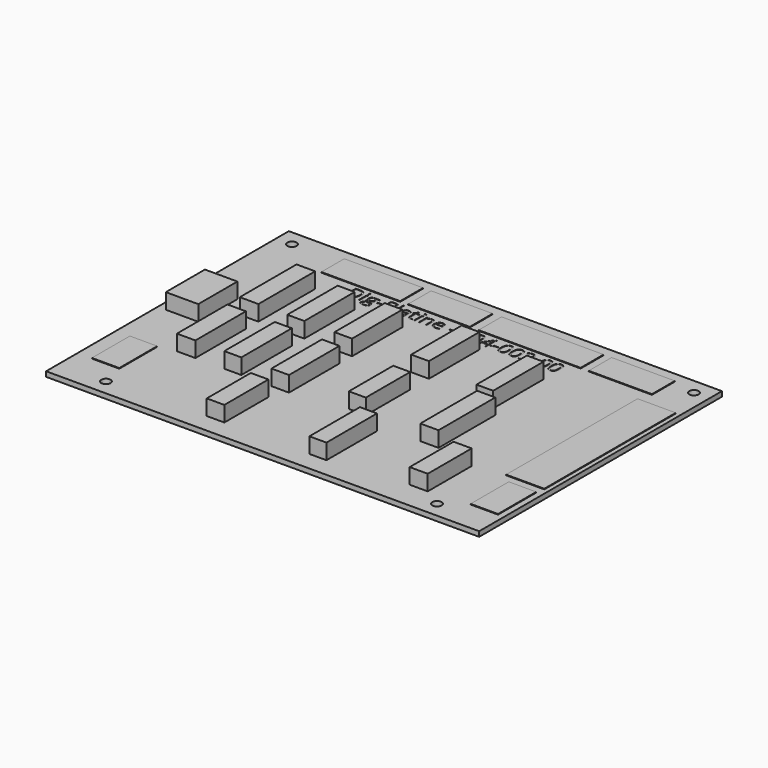
from build123d import *

# Parameters (mm, degrees)
F0_W         = 139.5791522491
F0_H         = 97.79
F0_R         = 1.5
F0_W_2       = 8.8093318045
F0_H_2       = 15.2748934925
F0_W_3       = 5.6705586612
F0_H_3       = 17.7562497556
F0_W_4       = 5.9523582458
F0_H_4       = 20.3446323285
F0_W_5       = 5.4862108082
F0_W_6       = 5.6576561183
F0_W_7       = 5.4957289249
F0_H_5       = 20.3665252775
F0_W_8       = 5.819004029
F0_H_6       = 17.6994800568
F0_W_9       = 8.8422298431
F0_H_7       = 15.3777878731
F0_W_10      = 5.4677436128
F0_H_8       = 17.8766759345
F0_W_11      = 5.862781778
F0_H_9       = 22.8744579945
F0_W_12      = 10.4659721255
F0_H_10      = 15.7669195905
F0_W_13      = 6.0005448759
F0_H_11      = 22.8592171334
F0_H_12      = 20.2875542454
F0_W_14      = 25.4173632711
F0_H_13      = 9.2426761985
F0_W_15      = 19.8445699643
F0_W_16      = 5.7087126188
F0_H_14      = 20.3202972189
F0_W_17      = 5.3689070046
F0_W_18      = 12.3022273183
F0_H_15      = 52.9572535306
F0_W_19      = 32.893058029
F0_W_20      = 20.3882530332
F1_DEPTH     = 1.6
F2_TEXT_SIZE = 6.1743944469
F3_DEPTH     = 0.1
F4_DEPTH     = 0.2
F5_DEPTH     = 5


# Not quite as in the source:
# - Text() gives the source's letters only with a copy of the font that has no kerning and outlines rounded to 1/6400 em; it was checked with that copy


with BuildPart() as f1:
    # F0 (on Top) → F1 (new body)
    with BuildSketch(Plane.XY):
        Rectangle(F0_W, F0_H)
        with Locations((-54.5495761246, -43.815)):
            Circle(F0_R, mode=Mode.SUBTRACT)
        with Locations((-60.6642495841, -28.6812912673)):
            Rectangle(F0_W_2, F0_H_2, mode=Mode.SUBTRACT)
        with Locations((-20.1366990805, -33.8139589876)):
            Rectangle(F0_W_3, F0_H_3, mode=Mode.SUBTRACT)
        with Locations((-47.9160919785, -9.6386900987)):
            Rectangle(F0_W_4, F0_H_4, mode=Mode.SUBTRACT)
        with Locations((-32.8816743568, -9.6386900987)):
            Rectangle(F0_W_5, F0_H_4, mode=Mode.SUBTRACT)
        with Locations((-17.594573088, -9.6386900987)):
            Rectangle(F0_W_6, F0_H_4, mode=Mode.SUBTRACT)
        with Locations((12.853551656, -32.5088212267)):
            Rectangle(F0_W_7, F0_H_5, mode=Mode.SUBTRACT)
        with Locations((52.1304238754, -43.815)):
            Circle(F0_R, mode=Mode.SUBTRACT)
        with Locations((43.2012882084, -31.1752967536)):
            Rectangle(F0_W_8, F0_H_6, mode=Mode.SUBTRACT)
        with Locations((63.4397342801, -31.1942892149)):
            Rectangle(F0_W_9, F0_H_7, mode=Mode.SUBTRACT)
        with Locations((5.2794092335, -8.4047119017)):
            Rectangle(F0_W_10, F0_H_8, mode=Mode.SUBTRACT)
        with Locations((30.4834870622, -8.3737772657)):
            Rectangle(F0_W_11, F0_H_9, mode=Mode.SUBTRACT)
        with Locations((-61.9684271514, 3.9792419411)):
            Rectangle(F0_W_12, F0_H_10, mode=Mode.SUBTRACT)
        with Locations((-47.9401852936, 17.0108985621)):
            Rectangle(F0_W_13, F0_H_11, mode=Mode.SUBTRACT)
        with Locations((-32.8816743568, 15.7250671182)):
            Rectangle(F0_W_5, F0_H_12, mode=Mode.SUBTRACT)
        with Locations((-17.594573088, 15.7250671182)):
            Rectangle(F0_W_6, F0_H_12, mode=Mode.SUBTRACT)
        with Locations((-64.7095761246, 43.815)):
            Circle(F0_R, mode=Mode.SUBTRACT)
        with Locations((-36.5455234423, 40.930185467)):
            Rectangle(F0_W_14, F0_H_13, mode=Mode.SUBTRACT)
        with Locations((-11.3320440287, 40.930185467)):
            Rectangle(F0_W_15, F0_H_13, mode=Mode.SUBTRACT)
        with Locations((5.1589247305, 18.2475312613)):
            Rectangle(F0_W_16, F0_H_14, mode=Mode.SUBTRACT)
        with Locations((28.0277524143, 15.7250671182)):
            Rectangle(F0_W_17, F0_H_12, mode=Mode.SUBTRACT)
        with Locations((62.2001700103, 5.6103980169)):
            Rectangle(F0_W_18, F0_H_15, mode=Mode.SUBTRACT)
        with Locations((17.8911256953, 40.930185467)):
            Rectangle(F0_W_19, F0_H_13, mode=Mode.SUBTRACT)
        with Locations((47.1142940223, 40.930185467)):
            Rectangle(F0_W_20, F0_H_13, mode=Mode.SUBTRACT)
        with Locations((64.8304238754, 43.815)):
            Circle(F0_R, mode=Mode.SUBTRACT)
        with Locations((-36.5455234423, 40.930185467)):
            Rectangle(F0_W_14, F0_H_13)
        with Locations((-11.3320440287, 40.930185467)):
            Rectangle(F0_W_15, F0_H_13)
        with Locations((17.8911256953, 40.930185467)):
            Rectangle(F0_W_19, F0_H_13)
        with Locations((47.1142940223, 40.930185467)):
            Rectangle(F0_W_20, F0_H_13)
        with Locations((-47.9401852936, 17.0108985621)):
            Rectangle(F0_W_13, F0_H_11)
        with Locations((-32.8816743568, 15.7250671182)):
            Rectangle(F0_W_5, F0_H_12)
        with Locations((-17.594573088, 15.7250671182)):
            Rectangle(F0_W_6, F0_H_12)
        with Locations((5.1589247305, 18.2475312613)):
            Rectangle(F0_W_16, F0_H_14)
        with Locations((28.0277524143, 15.7250671182)):
            Rectangle(F0_W_17, F0_H_12)
        with Locations((62.2001700103, 5.6103980169)):
            Rectangle(F0_W_18, F0_H_15)
        with Locations((-61.9684271514, 3.9792419411)):
            Rectangle(F0_W_12, F0_H_10)
        with Locations((-47.9160919785, -9.6386900987)):
            Rectangle(F0_W_4, F0_H_4)
        with Locations((-32.8816743568, -9.6386900987)):
            Rectangle(F0_W_5, F0_H_4)
        with Locations((-17.594573088, -9.6386900987)):
            Rectangle(F0_W_6, F0_H_4)
        with Locations((5.2794092335, -8.4047119017)):
            Rectangle(F0_W_10, F0_H_8)
        with Locations((30.4834870622, -8.3737772657)):
            Rectangle(F0_W_11, F0_H_9)
        with Locations((-60.6642495841, -28.6812912673)):
            Rectangle(F0_W_2, F0_H_2)
        with Locations((-20.1366990805, -33.8139589876)):
            Rectangle(F0_W_3, F0_H_3)
        with Locations((12.853551656, -32.5088212267)):
            Rectangle(F0_W_7, F0_H_5)
        with Locations((43.2012882084, -31.1752967536)):
            Rectangle(F0_W_8, F0_H_6)
        with Locations((63.4397342801, -31.1942892149)):
            Rectangle(F0_W_9, F0_H_7)
    extrude(amount=-F1_DEPTH)

    # F2 (on face) → F3 (cut)
    with BuildSketch(Plane.XY):
        with Locations((-37.6409441233, 30.5361393839)):
            Text('Dig-Platine - 304-003-00', F2_TEXT_SIZE, font='Open Sans', text_align=(TextAlign.LEFT, TextAlign.BOTTOM))
    extrude(amount=-F3_DEPTH, mode=Mode.SUBTRACT)

    # F0 (on Top) → F4 (join)
    with BuildSketch(Plane.XY):
        with Locations((-36.5455234423, 40.930185467)):
            Rectangle(F0_W_14, F0_H_13)
        with Locations((-11.3320440287, 40.930185467)):
            Rectangle(F0_W_15, F0_H_13)
        with Locations((17.8911256953, 40.930185467)):
            Rectangle(F0_W_19, F0_H_13)
        with Locations((47.1142940223, 40.930185467)):
            Rectangle(F0_W_20, F0_H_13)
        with Locations((62.2001700103, 5.6103980169)):
            Rectangle(F0_W_18, F0_H_15)
        with Locations((63.4397342801, -31.1942892149)):
            Rectangle(F0_W_9, F0_H_7)
        with Locations((-60.6642495841, -28.6812912673)):
            Rectangle(F0_W_2, F0_H_2)
    extrude(amount=F4_DEPTH)

    # F0 (on Top) → F5 (join)
    with BuildSketch(Plane.XY):
        with Locations((-47.9401852936, 17.0108985621)):
            Rectangle(F0_W_13, F0_H_11)
        with Locations((-32.8816743568, 15.7250671182)):
            Rectangle(F0_W_5, F0_H_12)
        with Locations((-17.594573088, 15.7250671182)):
            Rectangle(F0_W_6, F0_H_12)
        with Locations((5.1589247305, 18.2475312613)):
            Rectangle(F0_W_16, F0_H_14)
        with Locations((28.0277524143, 15.7250671182)):
            Rectangle(F0_W_17, F0_H_12)
        with Locations((-47.9160919785, -9.6386900987)):
            Rectangle(F0_W_4, F0_H_4)
        with Locations((-32.8816743568, -9.6386900987)):
            Rectangle(F0_W_5, F0_H_4)
        with Locations((-17.594573088, -9.6386900987)):
            Rectangle(F0_W_6, F0_H_4)
        with Locations((5.2794092335, -8.4047119017)):
            Rectangle(F0_W_10, F0_H_8)
        with Locations((30.4834870622, -8.3737772657)):
            Rectangle(F0_W_11, F0_H_9)
        with Locations((-20.1366990805, -33.8139589876)):
            Rectangle(F0_W_3, F0_H_3)
        with Locations((12.853551656, -32.5088212267)):
            Rectangle(F0_W_7, F0_H_5)
        with Locations((43.2012882084, -31.1752967536)):
            Rectangle(F0_W_8, F0_H_6)
        with Locations((-61.9684271514, 3.9792419411)):
            Rectangle(F0_W_12, F0_H_10)
    extrude(amount=F5_DEPTH)


solid = f1.part
